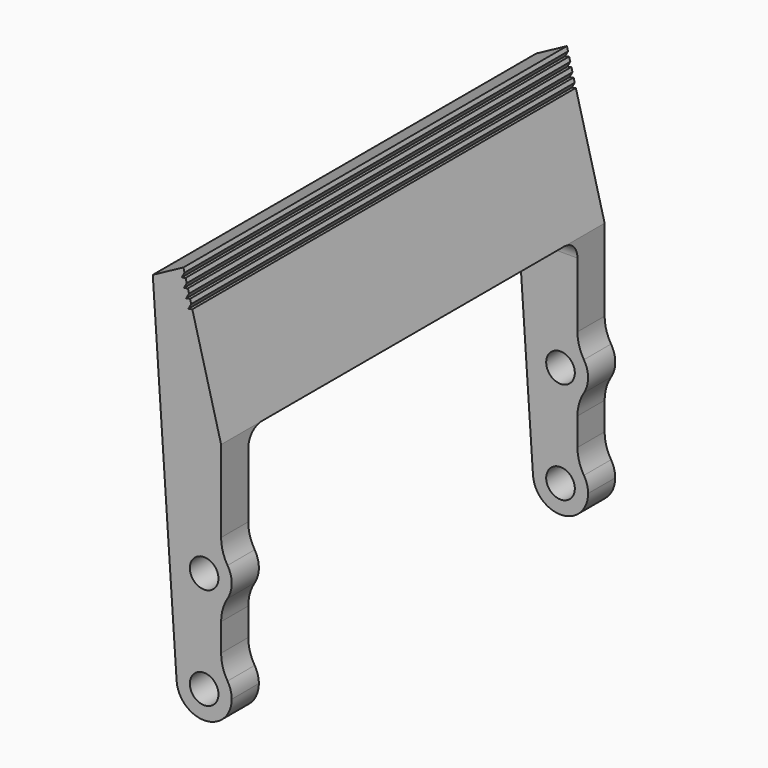
from build123d import *

# Parameters (mm, degrees)
F0_R     = 1.6875
F0_R_2   = 2
F1_DEPTH = 56.5
F3_START = -4
F3_DEPTH = 48.5
F5_R     = 5
F6_R     = 2


# Not quite as in the source:
# - a feature of the source that left no trace in its solid (it failed there, or was rolled back) is left out
# - a feature names something its author has since deleted; it is built from what else it names


with BuildPart() as f1:
    # F0 (on Front) → F1 (new body)
    with BuildSketch(Plane.XZ):
        with BuildLine():
            ThreePointArc((-3.2424633134, -0.2212050215), (-1.5238508153, 2.8706059801), (2, 2.5617376915))
            Line((2, 2.5617376915), (2, 9.4382623085))
            ThreePointArc((2, 9.4382623085), (3.25, 12), (2, 14.5617376915))
            Line((2, 14.5617376915), (2, 16))
            Line((2, 16), (2, 26.0145742767))
            Line((2, 26.0145742767), (-1.3932364987, 38.9411094094))
            Line((-1.3932364987, 38.9411094094), (-1.8768517883, 38.8141596092))
            Line((-1.8768517883, 38.8141596092), (-1.5244873121, 39.4411094094))
            Line((-1.5244873121, 39.4411094094), (-1.6557381254, 39.9411094094))
            Line((-1.6557381254, 39.9411094094), (-2.1393534149, 39.8141596092))
            Line((-2.1393534149, 39.8141596092), (-1.7869889387, 40.4411094094))
            Line((-1.7869889387, 40.4411094094), (-1.918239752, 40.9411094094))
            Line((-1.918239752, 40.9411094094), (-2.4018550415, 40.8141596092))
            Line((-2.4018550415, 40.8141596092), (-2.0494905653, 41.4411094094))
            Line((-2.0494905653, 41.4411094094), (-2.1807413786, 41.9411094094))
            Line((-2.1807413786, 41.9411094094), (-2.6643566681, 41.8141596092))
            Line((-2.6643566681, 41.8141596092), (-2.3119921919, 42.4411094094))
            Line((-2.3119921919, 42.4411094094), (-2.4432430052, 42.9411094094))
            Line((-2.4432430052, 42.9411094094), (-6.0546269865, 41))
            Line((-6.0546269865, 41), (-3.2424633134, -0.2212050215))
        make_face()
        with Locations((0, 12)):
            Circle(F0_R, mode=Mode.SUBTRACT)
        with BuildLine():
            ThreePointArc((3.25, 0), (2.9208303614, 1.4252192814), (2, 2.5617376915))
            ThreePointArc((2, 2.5617376915), (-1.5238508153, 2.8706059801), (-3.2424633134, -0.2212050215))
            ThreePointArc((-3.2424633134, -0.2212050215), (0.1106666878, -3.2481152819), (3.25, 0))
        make_face()
        Circle(F0_R_2, mode=Mode.SUBTRACT)
        Circle(F0_R_2)
        Circle(F0_R, mode=Mode.SUBTRACT)
    extrude(amount=F1_DEPTH)

    # F2 (on face) → F3 (cut)
    with BuildSketch(Plane(origin=(0, 0, 0), x_dir=(-1, 0, 0), z_dir=(0, 1, 0)).offset(F3_START)):
        with BuildLine():
            Line((5.032301952, 26.0145742767), (-2, 26.0145742767))
            Line((-2, 26.0145742767), (-2.5801925668, 13.9761341853))
            ThreePointArc((-2.5801925668, 13.9761341853), (-3.2462320816, 12.1564521408), (-2.7582721639, 10.2811530987))
            Line((-2.7582721639, 10.2811530987), (-3.2462320816, 0.1564521408))
            ThreePointArc((-3.2462320816, 0.1564521408), (-0.1888379833, -3.2445092412), (3.2424633134, -0.2212050215))
            Line((3.2424633134, -0.2212050215), (5.032301952, 26.0145742767))
        make_face()
    extrude(amount=-F3_DEPTH, mode=Mode.SUBTRACT)

    # F5
    f5_edges = [f1.edges().sort_by_distance(p)[0] for p in [
        (2, -2, 9.438262),
        (2, -54.5, 9.438262),
        (2, -2, 2.561738),
        (2, -2, 14.561738),
        (2, -54.5, 14.561738),
        (2, -54.5, 2.561738),
    ]]
    fillet(f5_edges, radius=F5_R)

    # F6
    f6_edges = [f1.edges().sort_by_distance(p)[0] for p in [
        (-1.516151, -52.5, 26.014574),
        (-1.516151, -4, 26.014574),
    ]]
    fillet(f6_edges, radius=F6_R)


solid = f1.part
